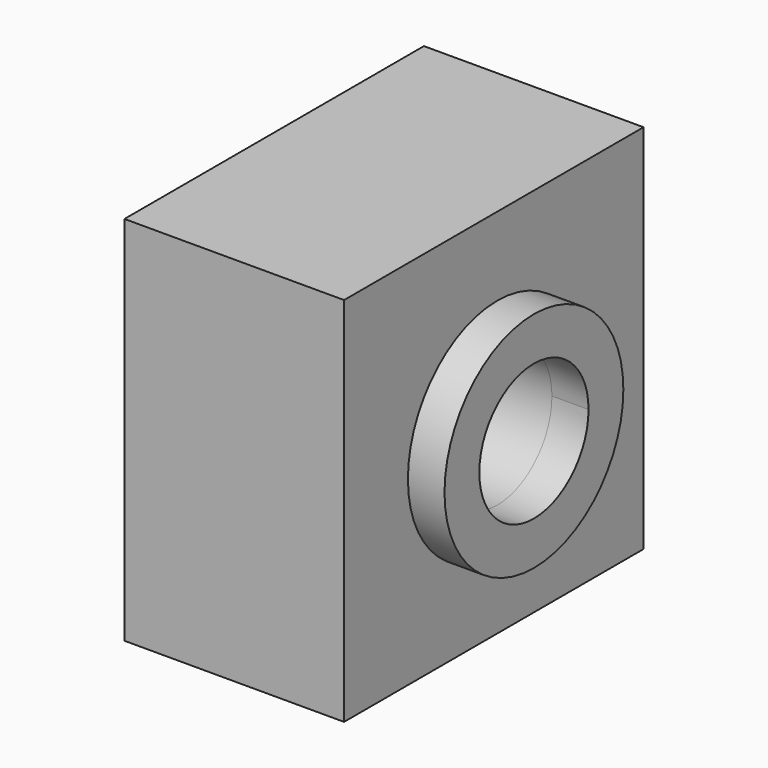
from build123d import *
from build123d import SkipClean  # not in build123d's __all__

# Parameters (mm, degrees)
F0_R     = 22.9010259121
F0_R_2   = 13.9818591187
F1_DEPTH = 30
F3_DEPTH = 22.5
F4_R     = 13.9818591187
F5_DEPTH = 52.501


with BuildPart() as f1:
    # F0 (on Right) → F1 (new body, symmetric)
    with BuildSketch(Plane.YZ):
        Circle(F0_R)
        Circle(F0_R_2, mode=Mode.SUBTRACT)
    extrude(amount=F1_DEPTH, both=True)

    # F2 (on Right) → F3 (join, symmetric)
    with BuildSketch(Plane.YZ):
        Polygon((37.4482907355, 38.9522351325), (0, 38.9522351325), (-39.253026247, 38.9522351325), (-39.253026247, -37.1474996209), (37.4482907355, -37.1474996209), align=None)
    extrude(amount=F3_DEPTH, both=True)

    # F4 (on face) → F5 (cut, through all)
    with BuildSketch(Plane(origin=(-22.5, 0, 0), x_dir=(0, -1, 0), z_dir=(-1, 0, 0))):
        Circle(F4_R)
    with SkipClean():  # cleaning this boolean's faces spoils the solid; the shape is the same uncleaned
        extrude(amount=-F5_DEPTH, mode=Mode.SUBTRACT)


solid = f1.part
